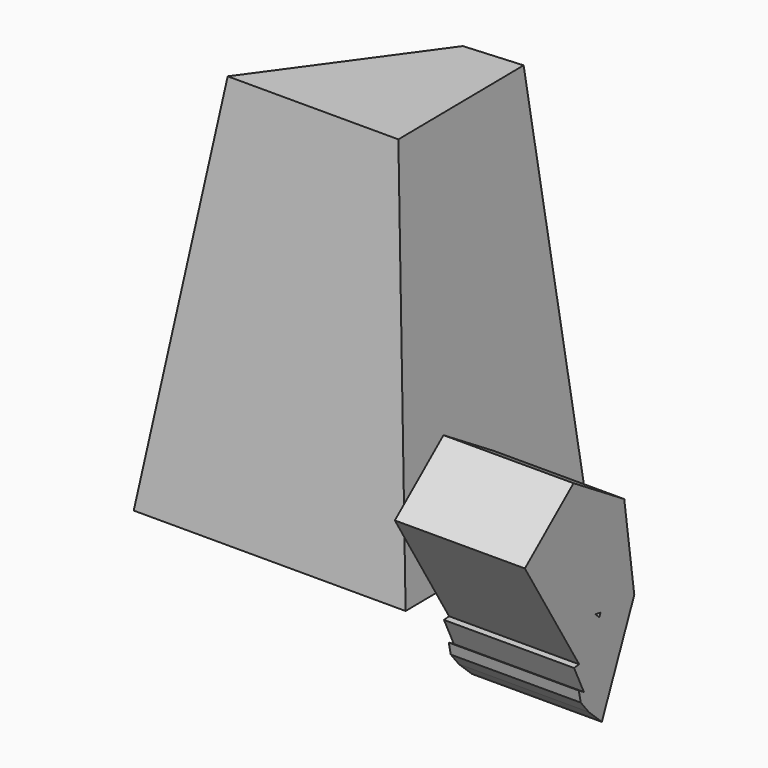
from build123d import *

# Parameters (mm, degrees)
F1_DEPTH = 76.2
F1_TAPER = 5
F3_DEPTH = 25.4


with BuildPart() as f1:
    # F0 (on Top) → F1 (new body)
    with BuildSketch(Plane.XY):
        Polygon((-22.784885, 18.140275), (-44.167623, 16.562859), (-75.365387, -26.728423), (-22.259081, -26.728423), align=None)
    extrude(amount=F1_DEPTH, taper=F1_TAPER)


with BuildPart() as f3:
    # F2 (on Right) → F3 (new body)
    with BuildSketch(Plane.YZ):
        Polygon((-38.391053, 1.171646), (-37.639222, 2.93949), (-43.934762, 13.332287), (-45.180503, 13.209712), (-42.774543, 8.101393), (-44.026013, 8.848615), (-43.529257, 6.582182), (-41.551817, 4.140794), align=None)
        Polygon((-43.934762, 13.332287), (-37.639222, 2.93949), (-36.464883, 5.700816), (-39.248545, 9.116296), (-41.390125, 13.582669), align=None)
        Polygon((-57.181932, 35.200968), (-43.934762, 13.332287), (-41.390125, 13.582669), (-41.192569, 13.602108), (-38.997059, 19.418651), (-37.323743, 17.879222), (-38.01373, 13.910294), (-35.63875, 11.307757), (-36.464883, 5.700816), (-30.471835, 19.792784), (-32.921135, 37.272938), (-45.306243, 45.027804), align=None)
        Polygon((-38.731471, 20.122271), (-38.997059, 19.418651), (-39.959099, 20.303715), align=None, mode=Mode.SUBTRACT)
        Polygon((-39.248545, 9.116296), (-36.464883, 5.700816), (-35.63875, 11.307757), (-38.01373, 13.910294), (-37.323743, 17.879222), (-38.997059, 19.418651), (-41.192569, 13.602108), (-41.390125, 13.582669), align=None)
    extrude(amount=F3_DEPTH)


solid = Compound([f1.part, f3.part])
